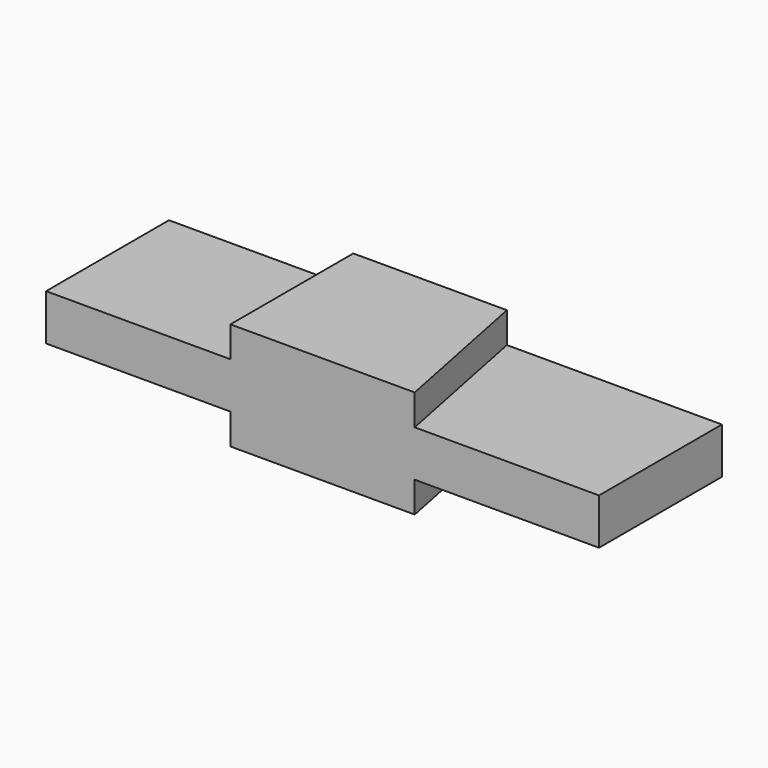
from build123d import *

# Parameters (mm, degrees)
F0_W     = 114.3
F0_H     = 31.75
F1_DEPTH = 11.1125
F2_W     = 38.1
F2_H     = 31.75
F3_DEPTH = 6.35
F5_DEPTH = 6.35


# Not quite as in the source:
# - a feature of the source that left no trace in its solid (it failed there, or was rolled back) is left out
# - a pattern or mirror of a feature is missing from the dataset's text; its kind, count and spacing are read off the source's solid


with BuildPart() as f1:
    # F0 (on Top) → F1 (new body, symmetric)
    with BuildSketch(Plane.XY):
        Rectangle(F0_W, F0_H)
    extrude(amount=F1_DEPTH, both=True)

    # F2 (on face) → F3 (cut)
    with BuildSketch(Plane.XY.offset(11.1125)):
        with Locations((-38.1, 0)):
            Rectangle(F2_W, F2_H)
    f3 = extrude(amount=-F3_DEPTH, mode=Mode.SUBTRACT)

    # F3_copies: F3 across plane
    add(f3.mirror(Plane(origin=(0, 0, 0), x_dir=(-1, 0, 0), z_dir=(0, 0, -1))), mode=Mode.SUBTRACT)

    # F4 (on face) → F5 (cut)
    with BuildSketch(Plane.XY.offset(11.1125)):
        Polygon((57.15, -15.875), (57.15, 15.875), (12.7, 15.875), (19.05, -15.875), align=None)
    f5 = extrude(amount=-F5_DEPTH, mode=Mode.SUBTRACT)

    # F5_copies: F5 across plane
    add(f5.mirror(Plane(origin=(0, 0, 0), x_dir=(-1, 0, 0), z_dir=(0, 0, -1))), mode=Mode.SUBTRACT)


solid = f1.part
